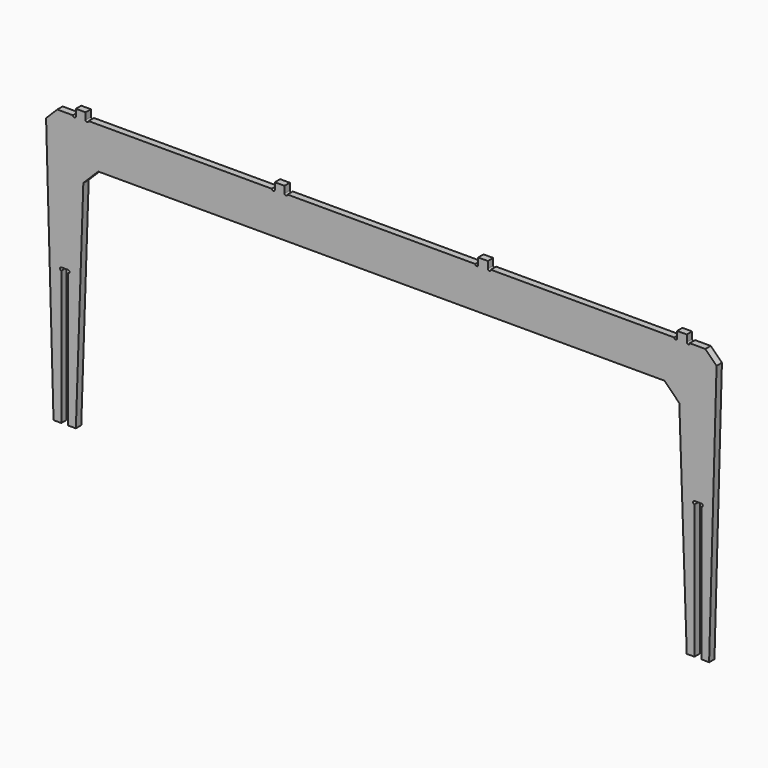
from build123d import *

# Parameters (mm, degrees)
F1_DEPTH = 18


# Not quite as in the source:
# - ends of sketch curves that miss each other by under 0.0002 mm in the source are joined


with BuildPart() as f1:
    # F0 (on Front) → F1 (new body)
    with BuildSketch(Plane.XZ):
        with BuildLine():
            Line((1444.9999982887, 361), (1444.9999982887, 379))
            Line((1444.9999982887, 379), (1418.9999982887, 379))
            Line((1418.9999982887, 379), (1418.9999982887, 361.0032042947))
            Line((1418.9999982887, 361.0032042947), (1418.9999982887, 361))
            ThreePointArc((1418.9999982887, 361), (1414.9978620926, 357.0032048651), (1410.9999984313, 361.0042723931))
            Line((1410.9999984313, 361.0042723931), (918.9999984313, 361.0042723931))
            ThreePointArc((918.9999984313, 361.0042723931), (914.9999984313, 357.0042723931), (910.9999984313, 361.0042723931))
            Line((910.9999984313, 361.0042723931), (910.9999984313, 379.0042723931))
            Line((910.9999984313, 379.0042723931), (884.9999984313, 379.0042723931))
            Line((884.9999984313, 379.0042723931), (884.9999984313, 361.0055952483))
            Line((884.9999984313, 361.0055952483), (884.9999984313, 361.0042723931))
            ThreePointArc((884.9999984313, 361.0042723931), (880.9986755762, 357.005595467), (876.9999986501, 361.0069181034))
            Line((876.9999986501, 361.0069181034), (372.9999978512, 361.1735978616))
            ThreePointArc((372.9999978512, 361.1735978616), (368.9986752099, 357.1749209454), (364.9999982887, 361.1762435819))
            Line((364.9999982887, 361.1762435819), (364.9999982887, 379.1762435819))
            Line((364.9999982887, 379.1762435819), (338.9999982887, 379.1762435819))
            Line((338.9999982887, 379.1762435819), (338.9999982887, 361.1783797782))
            ThreePointArc((338.9999982887, 361.1783797782), (334.9999982887, 357.1783797782), (330.9999982887, 361.1783797782))
            Line((330.9999982887, 361.1783797782), (-161.0000017113, 361.1783797782))
            ThreePointArc((-161.0000017113, 361.1783797782), (-165.0000017113, 357.1783797782), (-169.0000017113, 361.1783797782))
            Line((-169.0000017113, 361.1783797782), (-169.0000017113, 379.1783797782))
            Line((-169.0000017113, 379.1783797782), (-195.0000017113, 379.1783797782))
            Line((-195.0000017113, 379.1783797782), (-195.0000012844, 361.180516095))
            ThreePointArc((-195.0000012844, 361.180516095), (-198.9999999526, 357.1805172846), (-202.9999987156, 361.1805160001))
            Line((-202.9999987156, 361.1805160001), (-215.9862284595, 361.1805160001))
            Line((-215.9862284595, 361.1805160001), (-233.9862284595, 361.1805160001))
            Line((-233.9862284595, 361.1805160001), (-244.90749278, 361.1805160001))
            Line((-244.90749278, 361.1805160001), (-274.9862284595, 331.0746893941))
            Line((-274.9862284595, 331.0746893941), (-254.9862284595, -376.2833213137))
            Line((-254.9862284595, -376.2833213137), (-233.9862284595, -376.2833213137))
            Line((-233.9862284595, -376.2833213137), (-233.9862284595, -16.2833213137))
            ThreePointArc((-233.9862284595, -16.2833213137), (-237.9862284595, -12.2833213137), (-233.9862284595, -8.2833213137))
            Line((-233.9862284595, -8.2833213137), (-215.9862284595, -8.2833213137))
            ThreePointArc((-215.9862284595, -8.2833213137), (-211.9862284595, -12.2833213137), (-215.9862284595, -16.2833213137))
            Line((-215.9862284595, -16.2833213137), (-215.9862284595, -376.2833213137))
            Line((-215.9862284595, -376.2833213137), (-194.9862284595, -376.2833213137))
            Line((-194.9862284595, -376.2833213137), (-174.9862284595, 210.3365797868))
            Line((-174.9862284595, 210.3365797868), (-134.9862284595, 250.3365797868))
            Line((-134.9862284595, 250.3365797868), (1385.0137715405, 250.3365797868))
            Line((1385.0137715405, 250.3365797868), (1425.0137715405, 210.3365797868))
            Line((1425.0137715405, 210.3365797868), (1445.0137715405, -376.2833213137))
            Line((1445.0137715405, -376.2833213137), (1466.022162316, -375.6897371419))
            Line((1466.022162316, -375.6897371419), (1466.022162316, -15.6897371419))
            ThreePointArc((1466.022162316, -15.6897371419), (1462.0221624552, -11.6907923518), (1466.0200518963, -7.6897376986))
            Line((1466.0200518963, -7.6897376986), (1466.022162316, -7.6897371419))
            Line((1466.022162316, -7.6897371419), (1484.020051896, -7.6897371419))
            ThreePointArc((1484.020051896, -7.6897371419), (1488.020051896, -11.6897371419), (1484.020051896, -15.6897371419))
            Line((1484.020051896, -15.6897371419), (1484.020051896, -375.7643703854))
            Line((1484.020051896, -375.7643703854), (1505.0116611204, -376.3579545571))
            Line((1505.0116611204, -376.3579545571), (1525.0137715405, 331))
            Line((1525.0137715405, 331), (1494.9069982887, 361))
            Line((1494.9069982887, 361), (1466.022162316, 361))
            Line((1466.022162316, 361), (1452.9999982887, 361))
            ThreePointArc((1452.9999982887, 361), (1448.9999982887, 357), (1444.9999982887, 361))
        make_face()
    extrude(amount=F1_DEPTH)


solid = f1.part
